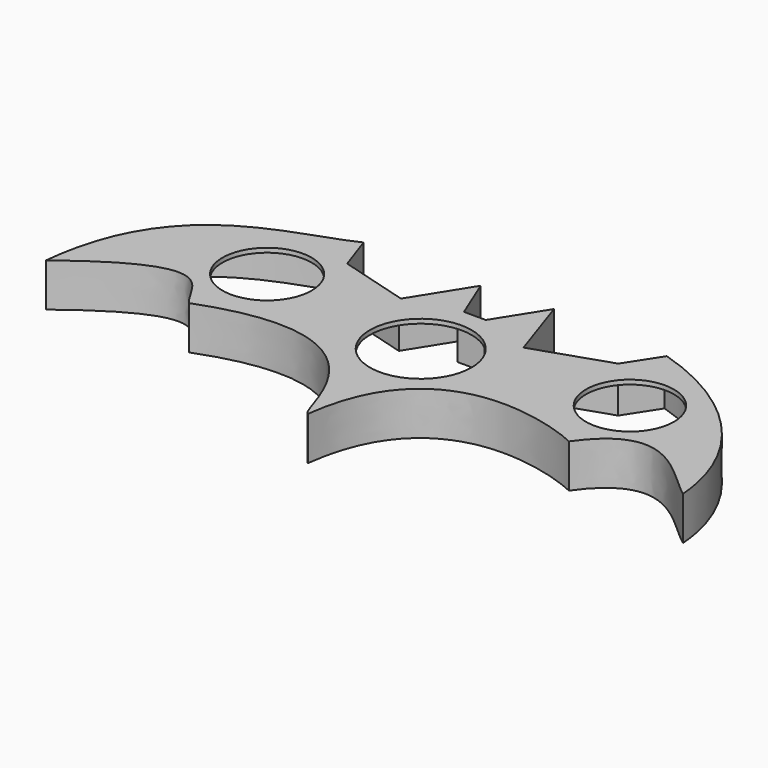
from build123d import *

# Parameters (mm, degrees)
F1_DEPTH = 10
F2_T     = -1
F3_R     = 10.2811491123
F3_R_2   = 10.1327379407
F3_R_3   = 11.7151578349
F4_DEPTH = 25


# Not quite as in the source:
# - a feature names something its author has since deleted; it is built from what else it names


with BuildPart() as f1:
    # F0 (on Top) → F1 (new body)
    with BuildSketch(Plane.XY):
        with BuildLine():
            Line((-31.0811921954, 14.660214074), (-33.9353941381, 22.9633450508))
            add(Edge.make_bspline(
                [(-33.9353941381, 22.9633450508), (-45.8711460233, 16.9954691082), (-70.7303881645, 15.644825995), (-74.2140114307, -18.1886926293)],
                knots=[0, 0, 0, 0, 57.5834804109, 57.5834804109, 57.5834804109, 57.5834804109], degree=3))
            add(Edge.make_bspline(
                [(-74.2140114307, -18.1886926293), (-47.157801188, 2.8172418051), (-47.8838291596, -11.176291999), (-43.6737610407, -15.1352264631)],
                knots=[0, 0, 0, 0, 30.6925161809, 30.6925161809, 30.6925161809, 30.6925161809], degree=3))
            add(Edge.make_bspline(
                [(-43.6737610407, -15.1352264631), (-3.7389839897, 0), (-2.5453862142, -35.4338922754), (0, -35.4338922754)],
                knots=[0, 0, 0, 0, 48.1604945698, 48.1604945698, 48.1604945698, 48.1604945698], degree=3))
            add(Edge.make_bspline(
                [(0, -35.4338922754), (4.5045536388, 0), (37.6610009838, -11.6567006335), (43.3694012463, -14.5109016448)],
                knots=[0, 0, 0, 0, 48.1526375331, 48.1526375331, 48.1526375331, 48.1526375331], degree=3))
            add(Edge.make_bspline(
                [(43.3694012463, -14.5109016448), (55.0884516883, 2.0732454632), (65.4413476586, -12.7122020349), (72.1837431192, -17.6538676023)],
                knots=[0, 0, 0, 0, 28.985246809, 28.985246809, 28.985246809, 28.985246809], degree=3))
            add(Edge.make_bspline(
                [(36.3872349262, 22.4479790777), (57.4458898787, 15.9976253073), (70.9220394555, 0), (72.1837431192, -17.6538676023)],
                knots=[0, 0, 0, 0, 53.754517075, 53.754517075, 53.754517075, 53.754517075], degree=3))
            Line((36.3872349262, 22.4479790777), (31.3764363527, 14.715090394))
            Line((31.3764363527, 14.715090394), (14.14907476, 8.932555189))
            Line((14.14907476, 8.932555189), (9.0551890513, 24.1082883068))
            Line((9.0551890513, 24.1082883068), (2.131328918, 13.103377074))
            add(Edge.make_bspline(
                [(-2.9128216118, 13.103377074), (-1.3559848446, 13.103377074), (0.5744921509, 13.103377074), (2.131328918, 13.103377074)],
                knots=[0, 0, 0, 0, 5.0441505298, 5.0441505298, 5.0441505298, 5.0441505298], degree=3))
            Line((-2.9128216118, 13.103377074), (-6.932257209, 22.9593385011))
            Line((-6.932257209, 22.9593385011), (-15.0030432269, 10.0596910343))
            Line((-15.0030432269, 10.0596910343), (-31.0811921954, 14.660214074))
        make_face()
    extrude(amount=F1_DEPTH)

    # F2
    f2_openings = [f1.faces().sort_by_distance(p)[0] for p in [
        (-1.663709, 0.488438, 0),
    ]]
    offset(amount=F2_T, openings=f2_openings, kind=Kind.INTERSECTION)

    # F3 (on face) → F4 (cut)
    with BuildSketch(Plane.XY.offset(10)):
        with Locations((-39.7835634649, 2.4649919942)):
            Circle(F3_R)
        with Locations((43.247744441, 3.2434102613)):
            Circle(F3_R_2)
        with Locations((0, -2.9839375056)):
            Circle(F3_R_3)
    extrude(amount=-F4_DEPTH, mode=Mode.SUBTRACT)


solid = f1.part
